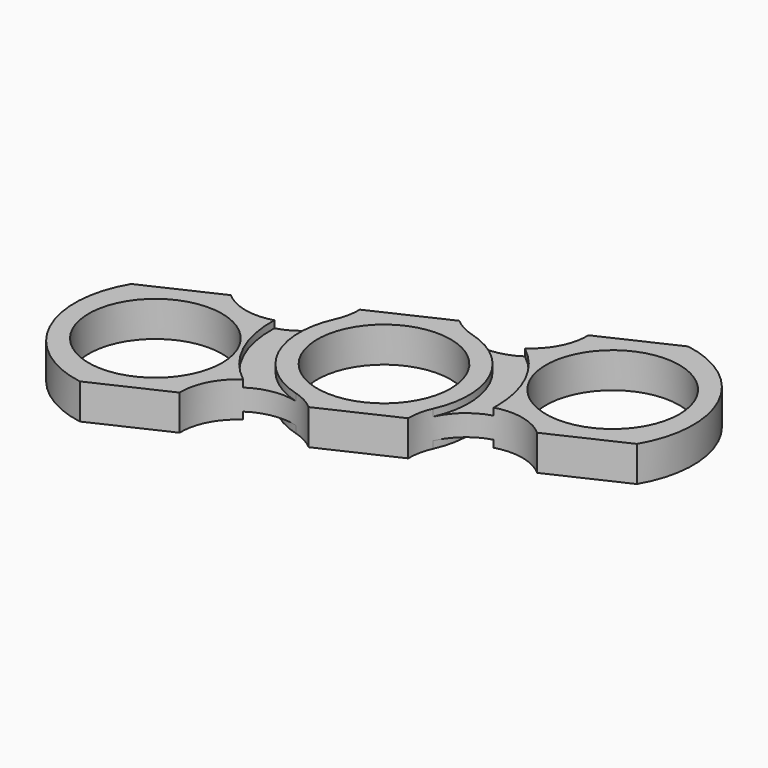
from build123d import *

# Parameters (mm, degrees)
F0_R          = 9.4365
F1_DEPTH      = 2.5
F1_DEPTH_BACK = 2.5
F2_R          = 9.4365
F3_DEPTH      = 1


# Not quite as in the source:
# - a pattern or mirror of a feature is missing from the dataset's text; its kind, count and spacing are read off the source's solid
# - a feature names something its author has since deleted; it is built from what else it names


with BuildPart() as f1:
    # F0 (on Top) → F1 (new body, two sides)
    with BuildSketch(Plane.XY) as f1_sk:
        with BuildLine():
            Line((-23.4990991809, 2.2827251198), (-33.7717440268, -2.5074878414))
            ThreePointArc((-33.7717440268, -2.5074878414), (-34.4396959074, -16.0594939461), (-23.628905745, -24.2588747303))
            Line((-23.628905745, -24.2588747303), (-13.3562608991, -19.4686617691))
            ThreePointArc((-13.3562608991, -19.4686617691), (-8.7397058477, -12.0182609074), (-0.0649032821, -13.270799925))
            Line((-0.0649032821, -13.270799925), (10.2077415638, -8.4805869639))
            ThreePointArc((10.2077415638, -8.4805869639), (14.8242966153, -1.0301861022), (23.4990991809, -2.2827251198))
            Line((23.4990991809, -2.2827251198), (33.7717440268, 2.5074878414))
            ThreePointArc((33.7717440268, 2.5074878414), (34.4396959074, 16.0594939461), (23.628905745, 24.2588747303))
            Line((23.628905745, 24.2588747303), (13.3562608991, 19.4686617691))
            ThreePointArc((13.3562608991, 19.4686617691), (8.7397058477, 12.0182609074), (0.0649032821, 13.270799925))
            Line((0.0649032821, 13.270799925), (-10.2077415638, 8.4805869639))
            ThreePointArc((-10.2077415638, 8.4805869639), (-14.8242966153, 1.0301861022), (-23.4990991809, 2.2827251198))
        make_face()
        with Locations((-23.564002463, -10.9880748053)):
            Circle(F0_R, mode=Mode.SUBTRACT)
        Circle(F0_R, mode=Mode.SUBTRACT)
        with Locations((23.564002463, 10.9880748053)):
            Circle(F0_R, mode=Mode.SUBTRACT)
    extrude(amount=F1_DEPTH)
    extrude(f1_sk.sketch, amount=-F1_DEPTH_BACK)

    # F2 (on face) → F3 (cut)
    with BuildSketch(Plane.XY.offset(2.5)):
        Circle(F2_R)
        with Locations((23.564002463, 10.9880748053)):
            Circle(F2_R)
        with Locations((-23.564002463, -10.9880748053)):
            Circle(F2_R)
        with BuildLine():
            ThreePointArc((-3.2152558613, -11.5612339197), (-10.8756934328, -5.0714191659), (-10.9231456523, 4.9683889802))
            ThreePointArc((-10.9231456523, 4.9683889802), (-12.9765670912, 2.225819641), (-15.9889787967, 0.5937651373))
            ThreePointArc((-15.9889787967, 0.5937651373), (-14.5009245926, -6.7618921879), (-9.8226669781, -12.6299332317))
            ThreePointArc((-9.8226669781, -12.6299332317), (-6.6360997478, -11.3713563932), (-3.2152558613, -11.5612339197))
        make_face()
        with BuildLine():
            ThreePointArc((3.2152559543, 11.5612338938), (9.5546604192, 7.2600595228), (12, 0))
            ThreePointArc((12, 0), (11.7276968614, -2.5418745694), (10.9231456122, -4.9683890683))
            ThreePointArc((10.9231456122, -4.9683890683), (12.9765670546, -2.2258196726), (15.9889787967, -0.5937651373))
            ThreePointArc((15.9889787967, -0.5937651373), (15.9972444619, -0.2969337069), (16, 0))
            ThreePointArc((16, 0), (14.3729376199, 7.0298409779), (9.8226669781, 12.6299332317))
            ThreePointArc((9.8226669781, 12.6299332317), (6.6360997955, 11.3713564009), (3.2152559543, 11.5612338938))
        make_face()
    f3 = extrude(amount=-F3_DEPTH, mode=Mode.SUBTRACT)

    # F3_copies: F3 across plane
    add(f3.mirror(Plane(origin=(0, 0, 0), x_dir=(-1, 0, 0), z_dir=(0, 0, -1))), mode=Mode.SUBTRACT)


solid = f1.part
